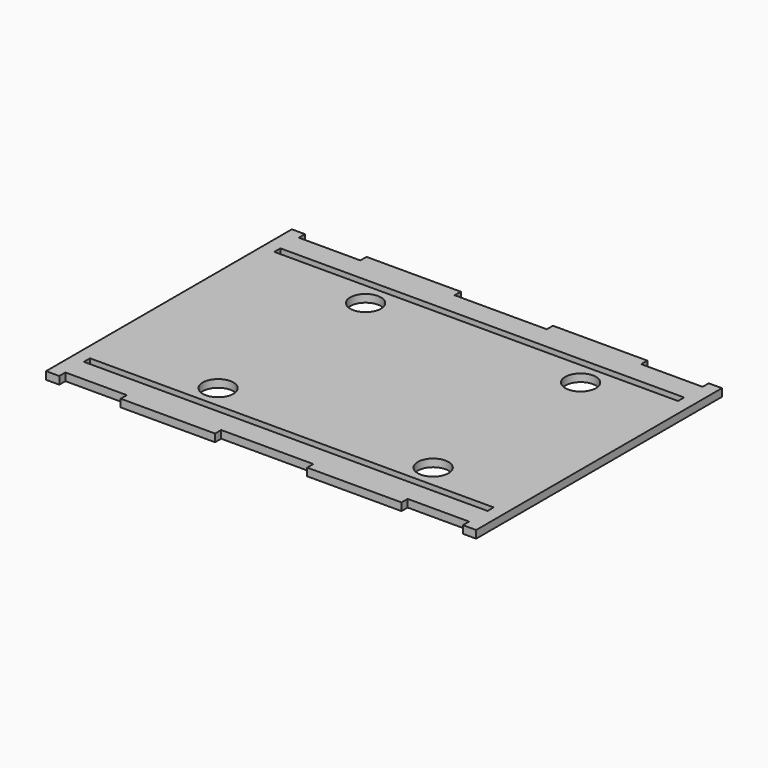
from build123d import *

# Parameters (mm, degrees)
F0_R     = 6.35
F1_DEPTH = 3.175


# Not quite as in the source:
# - a feature names something its author has since deleted; it is built from what else it names


with BuildPart() as f1:
    # F0 (on Top) → F1 (new body)
    with BuildSketch(Plane.XY):
        Polygon((-70.7512, 63.5), (-76.2, 63.5), (-76.2, -63.5), (-70.7512, -63.5), (-70.7512, -60.325), (-45.3512, -60.325), (-45.3512, -63.5), (-6.35, -63.5), (-6.35, -60.325), (31.75, -60.325), (31.75, -63.5), (70.7512, -63.5), (70.7512, -60.325), (96.1512, -60.325), (96.1512, -63.5), (101.6, -63.5), (101.6, 63.5), (96.1512, 63.5), (96.1512, 60.325), (70.7512, 60.325), (70.7512, 63.5), (31.75, 63.5), (31.75, 60.325), (-6.35, 60.325), (-6.35, 63.5), (-45.3512, 63.5), (-45.3512, 60.325), (-70.7512, 60.325), align=None)
        with Locations((-25.4, -38.1)):
            Circle(F0_R, mode=Mode.SUBTRACT)
        Polygon((-70.7512, -50.8), (-70.7512, -47.625), (-45.3512, -47.625), (-6.35, -47.625), (31.75, -47.625), (70.7512, -47.625), (96.1512, -47.625), (96.1512, -50.8), (70.7512, -50.8), (31.75, -50.8), (-6.35, -50.8), (-45.3512, -50.8), align=None, mode=Mode.SUBTRACT)
        with Locations((63.5, -38.1)):
            Circle(F0_R, mode=Mode.SUBTRACT)
        with Locations((-25.4, 38.1)):
            Circle(F0_R, mode=Mode.SUBTRACT)
        Polygon((96.1512, 50.8), (96.1512, 47.625), (70.7512, 47.625), (31.75, 47.625), (-6.35, 47.625), (-45.3512, 47.625), (-70.7512, 47.625), (-70.7512, 50.8), (-45.3512, 50.8), (-6.35, 50.8), (31.75, 50.8), (70.7512, 50.8), align=None, mode=Mode.SUBTRACT)
        with Locations((63.5, 38.1)):
            Circle(F0_R, mode=Mode.SUBTRACT)
    extrude(amount=F1_DEPTH)


solid = f1.part
